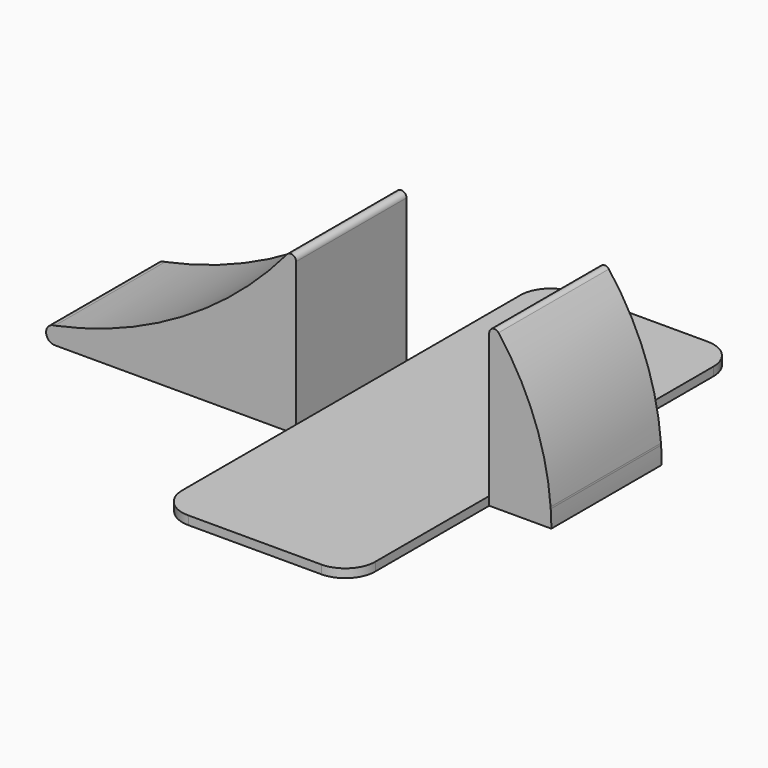
from build123d import *

# Parameters (mm, degrees)
F1_DEPTH = 50.8
F2_DEPTH = 114.3
F3_DEPTH = 63.5
F4_R     = 1.9065558253
F4_2_R   = 1.9065558253
F5_R     = 11.0377844072


with BuildPart() as f1:
    # F0 (on Front) → F1 (new body)
    with BuildSketch(Plane.XZ):
        with BuildLine():
            ThreePointArc((-124.4600042701, -24.3391744789), (-127.6350042701, -27.5141744789), (-124.4600042701, -30.6891744789))
            Line((-124.4600042701, -30.6891744789), (-124.4600042701, -24.3391744789))
        make_face()
        with BuildLine():
            Line((-124.4600042701, -30.6891744789), (-35.409415784, -30.6891744789))
            Line((-35.409415784, -30.6891744789), (-35.5600006878, -27.5141744789))
            Line((-35.5600006878, -27.5141744789), (-35.5600006878, -24.3391744789))
            Line((-35.5600006878, -24.3391744789), (-35.5600006878, 30.6891744789))
            ThreePointArc((-35.5600006878, 30.6891744789), (-75.1282903874, -4.7115572136), (-124.4600042701, -24.3391744789))
            Line((-124.4600042701, -24.3391744789), (-124.4600042701, -30.6891744789))
        make_face()
    extrude(amount=F1_DEPTH)

    # F4
    f4_edges = [f1.edges().sort_by_distance(p)[0] for p in [
        (-35.560001, -25.4, 30.689174),
    ]]
    fillet(f4_edges, radius=F4_R)


with BuildPart() as f1b:
    # F0 (on Front) → F1, piece 2 (new body)
    with BuildSketch(Plane.XZ):
        with BuildLine():
            Line((35.5599969625, -27.5141744789), (35.5599969625, -30.6891744789))
            Line((35.5599969625, -30.6891744789), (58.42, -30.6891744789))
            ThreePointArc((58.42, -30.6891744789), (58.3662051014, -27.5123531227), (58.2048820896, -24.3391744789))
            ThreePointArc((58.2048820896, -24.3391744789), (58.1831610583, -24.0266804729), (58.1603968933, -23.7142607236))
            ThreePointArc((58.1603968933, -23.7142607236), (51.2405848867, 5.3071676983), (35.5599969625, 30.6891744789))
            Line((35.5599969625, 30.6891744789), (35.5599969625, -24.3391744789))
            Line((35.5599969625, -24.3391744789), (35.5599969625, -27.5141744789))
        make_face()
    extrude(amount=F1_DEPTH)

    # F4#2
    f4_2_edges = [f1b.edges().sort_by_distance(p)[0] for p in [
        (35.559997, -25.4, 30.689174),
    ]]
    fillet(f4_2_edges, radius=F4_2_R)


with BuildPart() as f2:
    # F0 (on Front) → F2 (new body)
    with BuildSketch(Plane.XZ):
        Polygon((-33.02, -30.6891744789), (33.02, -30.6891744789), (35.5599969625, -30.6891744789), (35.5599969625, -27.5141744789), (-35.5600006878, -27.5141744789), (-35.409415784, -30.6891744789), align=None)
    extrude(amount=F2_DEPTH)

    # F0 (on Front) → F3 (join)
    with BuildSketch(Plane.XZ):
        Polygon((-33.02, -30.6891744789), (33.02, -30.6891744789), (35.5599969625, -30.6891744789), (35.5599969625, -27.5141744789), (-35.5600006878, -27.5141744789), (-35.409415784, -30.6891744789), align=None)
    extrude(amount=-F3_DEPTH)

    # F5
    f5_edges = [f2.edges().sort_by_distance(p)[0] for p in [
        (-35.484708, -114.3, -29.101674),
        (35.559997, -114.3, -29.101674),
        (35.559997, 63.5, -29.101674),
        (-35.484708, 63.5, -29.101674),
    ]]
    fillet(f5_edges, radius=F5_R)


solid = Compound([f1.part, f1b.part, f2.part])
